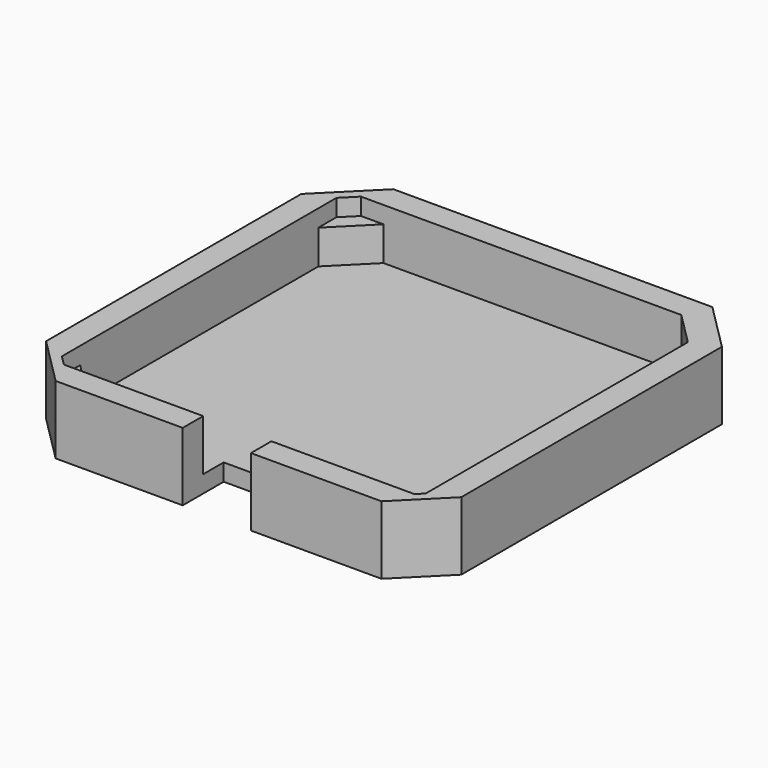
from build123d import *

# Parameters (mm, degrees)
F1_DEPTH     = 1
F3_DEPTH     = 3
F4_W         = 3.4
F4_H         = 3
F5_DEPTH     = 5
F7_DEPTH     = 1
F8_TEXT_SIZE = 20.2137905742
F9_DEPTH     = 0.5
F10_W        = 4
F10_H        = 3
F11_DEPTH    = 5


# Not quite as in the source:
# - Text() gives the source's letters only with a copy of the font that has no kerning and outlines rounded to 1/6400 em; it was checked with that copy


with BuildPart() as f1:
    # F0 (on Top) → F1 (new body)
    with BuildSketch(Plane.XY):
        Polygon((9.45, 12.25), (-9.25, 12.25), (-12.25, 9.25), (-12.25, -9.45), (-9.45, -12.25), (9.65, -12.25), (12.25, -9.65), (12.25, 9.45), align=None)
    extrude(amount=-F1_DEPTH)

    # F2 (on face) → F3 (join)
    with BuildSketch(Plane.XY):
        Polygon((12.25, 9.45), (9.45, 12.25), (-9.25, 12.25), (-12.25, 9.25), (-12.25, -9.45), (-9.45, -12.25), (9.65, -12.25), (12.25, -9.65), align=None)
        Polygon((-10.75, 8.6286796564), (-8.6286796564, 10.75), (8.8286796564, 10.75), (10.75, 8.8286796564), (10.75, -9.0286796564), (9.0286796564, -10.75), (-8.8286796564, -10.75), (-10.75, -8.8286796564), align=None, mode=Mode.SUBTRACT)
    extrude(amount=F3_DEPTH)

    # F4 (on face) → F5 (cut)
    with BuildSketch(Plane.XZ.offset(12.25)):
        with Locations((0, 1.5)):
            Rectangle(F4_W, F4_H)
    extrude(amount=-F5_DEPTH, mode=Mode.SUBTRACT)

    # F6 (on face) → F7 (cut)
    with BuildSketch(Plane.XY.offset(3)):
        Polygon((10.75, -9.0286796564), (9.0286796564, -10.75), (10.3815821931, -10.75), (10.75, -10.382595472), align=None)
        Polygon((-8.8286796564, -10.75), (-10.75, -8.8286796564), (-10.75, -10.175713338), (-10.1607451215, -10.75), align=None)
        Polygon((-10.75, 8.6286796564), (-8.6286796564, 10.75), (-9.9508352578, 10.75), (-10.75, 9.9508352578), align=None)
    extrude(amount=-F7_DEPTH, mode=Mode.SUBTRACT)

    # F8 (on face) → F9 (cut)
    with BuildSketch(Plane(origin=(0, 0, -1), x_dir=(1, 0, 0), z_dir=(0, 0, -1))):
        with Locations((-9.1125881299, -7.0895170793)):
            Text('Ti', F8_TEXT_SIZE, font='Open Sans', font_style=FontStyle.BOLD, text_align=(TextAlign.LEFT, TextAlign.BOTTOM))
    extrude(amount=-F9_DEPTH, mode=Mode.SUBTRACT)

    # F10 (on face) → F11 (cut)
    with BuildSketch(Plane(origin=(0, 0, -1), x_dir=(1, 0, 0), z_dir=(0, 0, -1))):
        with Locations((0, 10.75)):
            Rectangle(F10_W, F10_H)
    extrude(amount=-F11_DEPTH, mode=Mode.SUBTRACT)


solid = f1.part
